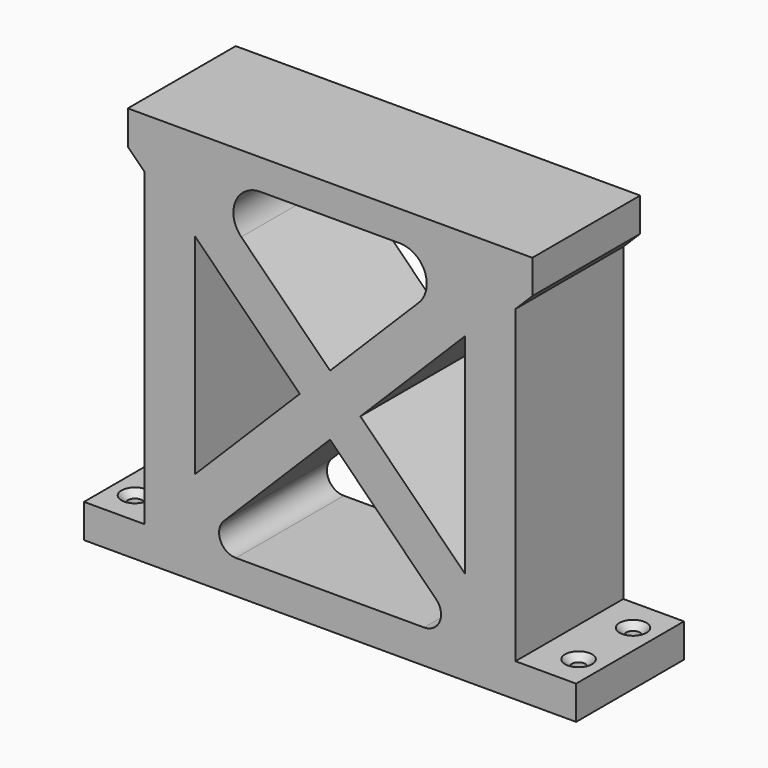
from build123d import *

# Parameters (mm, degrees)
F1_DEPTH       = 40
F2_R           = 8
F3_R           = 5
F5_D           = 4.2
F5_CSINK_D     = 8
F5_CSINK_ANGLE = 90
F6_SIZE        = 4.99999


# Not quite as in the source:
# - a fillet or chamfer is up to 0.001 mm smaller than in the source, because OpenCascade refuses the exact size


with BuildPart() as f1:
    # F0 (on Front) → F1 (new body)
    with BuildSketch(Plane.XZ):
        Polygon((-73, 10), (-73, 0), (0, 0), (73, 0), (73, 10), (55, 10), (55, 107), (60, 107), (60, 117), (0, 117), (-60, 117), (-60, 107), (-55, 107), (-55, 10), align=None)
        Polygon((0, 10), (-40, 10), (0, 50), (40, 10), align=None, mode=Mode.SUBTRACT)
        Polygon((-9, 59), (-40, 28), (-40, 90), align=None, mode=Mode.SUBTRACT)
        Polygon((40, 90), (40, 28), (9, 59), align=None, mode=Mode.SUBTRACT)
        Polygon((40, 108), (0, 68), (-40, 108), (0, 108), align=None, mode=Mode.SUBTRACT)
    extrude(amount=F1_DEPTH)

    # F2
    f2_edges = [f1.edges().sort_by_distance(p)[0] for p in [
        (-40, -20, 108),
        (40, -20, 108),
    ]]
    fillet(f2_edges, radius=F2_R)

    # F3
    f3_edges = [f1.edges().sort_by_distance(p)[0] for p in [
        (-40, -20, 10),
        (40, -20, 10),
    ]]
    fillet(f3_edges, radius=F3_R)

    # F5 (through all)
    with Locations(Plane.XY.offset(10)):
        with Locations((-65.8, -9.9), (-65.8, -30.1), (65.8, -30.1), (65.8, -9.9)):
            CounterSinkHole(F5_D / 2, F5_CSINK_D / 2, counter_sink_angle=F5_CSINK_ANGLE)

    # F6 (size 5 in the source; OpenCascade refuses exactly that, so slightly less here)
    f6_edges = [f1.edges().sort_by_distance(p)[0] for p in [
        (-55, -20, 107),
        (55, -20, 107),
    ]]
    chamfer(f6_edges, length=F6_SIZE)


solid = f1.part
